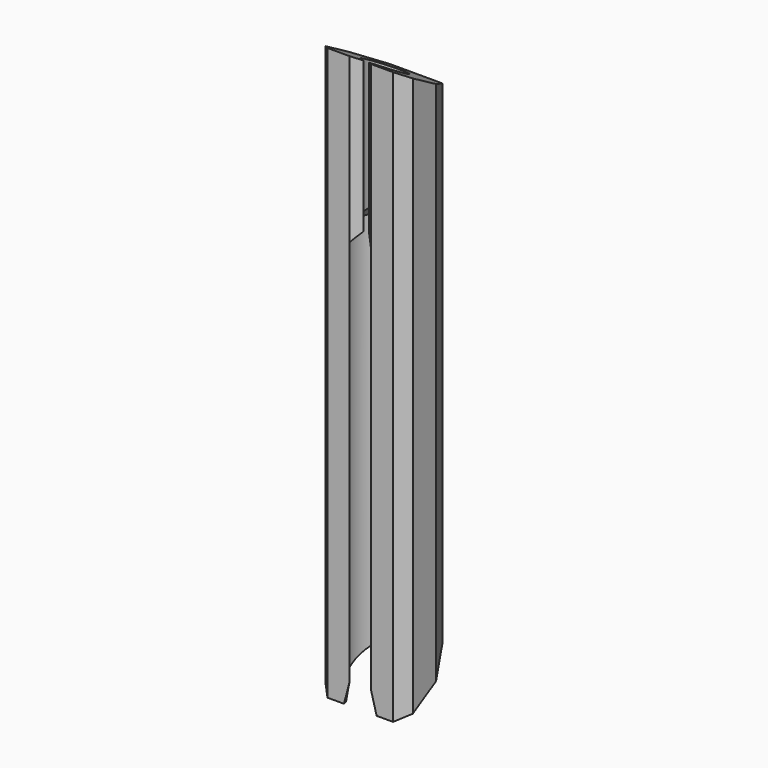
from build123d import *

# Parameters (mm, degrees)
F1_DEPTH  = 20
F2_DEPTH  = 15
F3_W      = 8
F3_H      = 0.1715728753
F4_DEPTH  = 35.001
F6_DEPTH  = 15
F7_SIZE   = 1.24999
F8_DEPTH  = 7.9
F9_W      = 8
F9_H      = 6.8284271247
F10_DEPTH = 3
F13_DEPTH = 3
F15_DEPTH = 8.001
F17_DEPTH = 60.901
F19_DEPTH = 8.001
F20_SIZE  = 1
F21_SIZE  = 0.5


# Not quite as in the source:
# - a fillet or chamfer is up to 0.001 mm smaller than in the source, because OpenCascade refuses the exact size


with BuildPart() as f1:
    # F0 (on Top) → F1 (new body)
    with BuildSketch(Plane.XY):
        with BuildLine():
            ThreePointArc((-1, -2.8284271247), (0, 3), (1, -2.8284271247))
            Line((1, -2.8284271247), (1, -3))
            Line((1, -3), (4, -3))
            Line((4, -3), (4, 4))
            Line((4, 4), (0, 4))
            Line((0, 4), (-4, 4))
            Line((-4, 4), (-4, -3))
            Line((-4, -3), (-1, -3))
            Line((-1, -3), (-1, -2.8284271247))
        make_face()
    extrude(amount=F1_DEPTH)

    # F2 (add): a face of the model
    f2_faces = [f1.faces().sort_by_distance(p)[0] for p in [
        (0, 3.1063014581, 20),
    ]]
    extrude(f2_faces, amount=F2_DEPTH)

    # F3 (on face) → F4 (cut, through all)
    with BuildSketch(Plane.XY.offset(35)):
        with Locations((0, -2.9142135624)):
            Rectangle(F3_W, F3_H)
    extrude(amount=-F4_DEPTH, mode=Mode.SUBTRACT)

    # F5 (on face) → F6 (join)
    with BuildSketch(Plane.XY.offset(35)):
        with BuildLine():
            ThreePointArc((-1, -1.4361406616), (0, 1.75), (1, -1.4361406616))
            Line((1, -1.4361406616), (0.25, -2.1322838932))
            Line((0.25, -2.1322838932), (1, -2.8284271247))
            Line((1, -2.8284271247), (4, -2.8284271247))
            Line((4, -2.8284271247), (4, 4))
            Line((4, 4), (-4, 4))
            Line((-4, 4), (-4, -2.8284271247))
            Line((-4, -2.8284271247), (-1, -2.8284271247))
            Line((-1, -2.8284271247), (-0.25, -2.1322838932))
            Line((-0.25, -2.1322838932), (-1, -1.4361406616))
        make_face()
    extrude(amount=F6_DEPTH)

    # F7 (size 1.25 in the source; OpenCascade refuses exactly that, so slightly less here)
    f7_edges = [f1.edges().sort_by_distance(p)[0] for p in [
        (0, 1.75, 35),
    ]]
    chamfer(f7_edges, length=F7_SIZE)

    # F8 (add): a face of the model
    f8_faces = [f1.faces().sort_by_distance(p)[0] for p in [
        (-2.5, -2.7232475559, 0),
    ]]
    extrude(f8_faces, amount=F8_DEPTH)

    # F9 (on face) → F10 (join)
    with BuildSketch(Plane(origin=(0, 0, -7.9), x_dir=(1, 0, 0), z_dir=(0, 0, -1))):
        with Locations((0, -0.5857864376)):
            Rectangle(F9_W, F9_H)
    extrude(amount=F10_DEPTH)

    # F12 (on face) → F13 (cut)
    with BuildSketch(Plane.XZ.offset(2.8284271247)):
        Polygon((0, 3.2961524227), (-3, -7.9), (1, -7.9), (3, -7.9), align=None)
    extrude(amount=-F13_DEPTH, mode=Mode.SUBTRACT)

    # F14 (on face) → F15 (cut, through all)
    with BuildSketch(Plane(origin=(-4, 0, 0), x_dir=(0, -1, 0), z_dir=(-1, 0, 0))):
        Polygon((-4, 46.0576057614), (2.8284271247, 50), (-4, 50), align=None)
    extrude(amount=-F15_DEPTH, mode=Mode.SUBTRACT)

    # F16 (on face) → F17 (cut, through all)
    with BuildSketch(Plane(origin=(0, 0, -10.9), x_dir=(1, 0, 0), z_dir=(0, 0, -1))):
        Polygon((4, -0.8309159426), (2.1703284663, -4), (4, -4), align=None)
        Polygon((-2.1703284663, -4), (-4, -0.8309159426), (-4, -4), align=None)
    extrude(amount=-F17_DEPTH, mode=Mode.SUBTRACT)

    # F18 (on face) → F19 (cut, through all)
    with BuildSketch(Plane.YZ.offset(4)):
        Polygon((4, 1.6660254038), (-2.8284271247, -2.2763688348), (-2.8284271247, -10.9), (4, -10.9), align=None)
    extrude(amount=-F19_DEPTH, mode=Mode.SUBTRACT)

    # F20
    f20_edges = [f1.edges().sort_by_distance(p)[0] for p in [
        (-4, -2.828427, 23.861816),
        (4, -2.828427, 23.861816),
    ]]
    chamfer(f20_edges, length=F20_SIZE)

    # F21
    f21_edges = [f1.edges().sort_by_distance(p)[0] for p in [
        (-2.170328, 4, 23.861816),
        (0, 4, 46.057606),
        (2.170328, 4, 23.861816),
        (0, 4, 1.666025),
    ]]
    chamfer(f21_edges, length=F21_SIZE)


solid = f1.part
